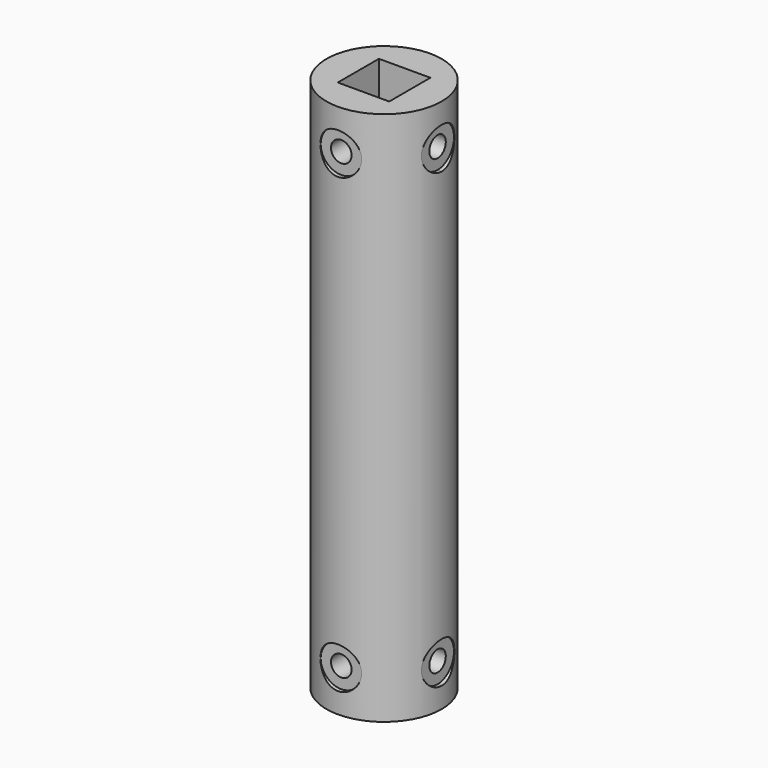
from build123d import *

# Parameters (mm, degrees)
F0_R            = 14
F0_W            = 12.5
F0_H            = 12.5
F1_DEPTH        = 130
F2_R            = 2.5
F4_DEPTH        = 25
F3_R            = 2.5
F5_DEPTH        = 25
F9_DEPTH        = 1
F9_COPIES_COUNT = 3
F9_COPIES_ANGLE = 180
F12_R           = 5
F13_DEPTH       = 1


# Not quite as in the source:
# - a pattern or mirror of a feature is missing from the dataset's text; its kind, count and spacing are read off the source's solid


with BuildPart() as f1:
    # F0 (on Top) → F1 (new body)
    with BuildSketch(Plane.XY):
        Circle(F0_R)
        Rectangle(F0_W, F0_H, mode=Mode.SUBTRACT)
    extrude(amount=F1_DEPTH)

    # F2 (on face) → F4 (cut, symmetric)
    with BuildSketch(Plane.XZ.offset(-6.25)):
        with Locations((0, 10)):
            Circle(F2_R)
        with Locations((0, 120)):
            Circle(F2_R)
    extrude(amount=F4_DEPTH, both=True, mode=Mode.SUBTRACT)

    # F3 (on face) → F5 (cut, symmetric)
    with BuildSketch(Plane.YZ.offset(-6.25)):
        with BuildLine():
            ThreePointArc((2.5, 120), (1.767766953, 121.767766953), (0, 122.5))
            ThreePointArc((0, 122.5), (-1.767766953, 118.232233047), (2.5, 120))
        make_face()
        with Locations((0, 10)):
            Circle(F3_R)
    extrude(amount=F5_DEPTH, both=True, mode=Mode.SUBTRACT)

    # F8 (on line) → F9 (cut)
    with BuildSketch(Plane(origin=(14, 0, 0), x_dir=(0, -1, 0), z_dir=(-1, 0, 0))):
        with BuildLine():
            ThreePointArc((5, 120), (3.5355339059, 123.5355339059), (0, 125))
            Line((0, 125), (0, 115))
            ThreePointArc((0, 115), (3.5355339059, 116.4644660941), (5, 120))
        make_face()
        with BuildLine():
            ThreePointArc((5, 10), (3.5355339059, 13.5355339059), (0, 15))
            Line((0, 15), (0, 5))
            ThreePointArc((0, 5), (3.5355339059, 6.4644660941), (5, 10))
        make_face()
        with BuildLine():
            Line((0, 5), (0, 15))
            ThreePointArc((0, 15), (-5, 10), (0, 5))
        make_face()
        with BuildLine():
            Line((0, 115), (0, 125))
            ThreePointArc((0, 125), (-5, 120), (0, 115))
        make_face()
    f9 = extrude(amount=F9_DEPTH, mode=Mode.SUBTRACT)

    # F9_copies: F9 ×3 about axis
    f9_copies_axis = Axis((0, 0, 0), (0, 0, 1))
    for i in range(1, F9_COPIES_COUNT):
        add(f9.rotate(f9_copies_axis, i * F9_COPIES_ANGLE / (F9_COPIES_COUNT - 1)), mode=Mode.SUBTRACT)

    # F12 (on line) → F13 (cut)
    with BuildSketch(Plane(origin=(0, -14, 0), x_dir=(-1, 0, 0), z_dir=(0, 1, 0))):
        with BuildLine():
            ThreePointArc((0, 125), (-3.5355339059, 116.4644660941), (5, 120))
            ThreePointArc((5, 120), (3.5355339059, 123.5355339059), (0, 125))
        make_face()
        with Locations((0, 10)):
            Circle(F12_R)
    extrude(amount=F13_DEPTH, mode=Mode.SUBTRACT)


solid = f1.part
